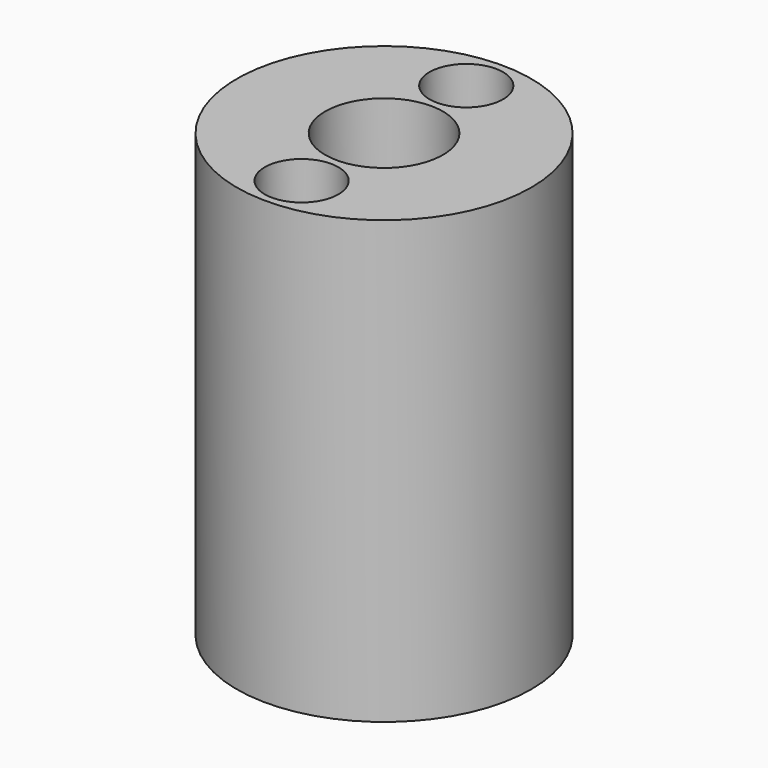
from build123d import *

# Parameters (mm, degrees)
F0_R      = 6.35
F1_DEPTH  = 19.05
F3_D      = 5.08
F8_D      = 3.175
F8_DEPTH  = 2.54
F8_TIP    = 0.9538662327
F9_D      = 3.175
F9_DEPTH  = 2.54
F9_TIP    = 0.9538662327
F11_D     = 11.938
F11_DEPTH = 12.7
F11_TIP   = 3.586537035


# Not quite as in the source:
# - the program builds the solid bodies; features that only make, move or delete a surface that nothing else refers to are left out


with BuildPart() as f1:
    # F0 (on Top) → F1 (new body)
    with BuildSketch(Plane.XY):
        Circle(F0_R)
    extrude(amount=F1_DEPTH)

    # F3 (through all)
    with Locations(Plane(origin=(0, 0, 0), x_dir=(1, 0, 0), z_dir=(0, 0, -1))):
        with Locations((0, 0)):
            Hole(F3_D / 2)

    # F8
    with Locations(Plane.XY.offset(19.05)):
        with Locations((0, 4.4337138534)):
            Hole(F8_D / 2, depth=F8_DEPTH)
            with Locations((0, 0, -(F8_DEPTH + F8_TIP / 2))):  # 118° drill point
                Cone(0, F8_D / 2, F8_TIP, mode=Mode.SUBTRACT)

    # F9
    with Locations(Plane.XY.offset(19.05)):
        with Locations((0, -4.445)):
            Hole(F9_D / 2, depth=F9_DEPTH)
            with Locations((0, 0, -(F9_DEPTH + F9_TIP / 2))):  # 118° drill point
                Cone(0, F9_D / 2, F9_TIP, mode=Mode.SUBTRACT)

    # F11
    with Locations(Plane(origin=(0, 0, 0), x_dir=(1, 0, 0), z_dir=(0, 0, -1))):
        with Locations((0, 0)):
            Hole(F11_D / 2, depth=F11_DEPTH)
            with Locations((0, 0, -(F11_DEPTH + F11_TIP / 2))):  # 118° drill point
                Cone(0, F11_D / 2, F11_TIP, mode=Mode.SUBTRACT)


solid = f1.part
